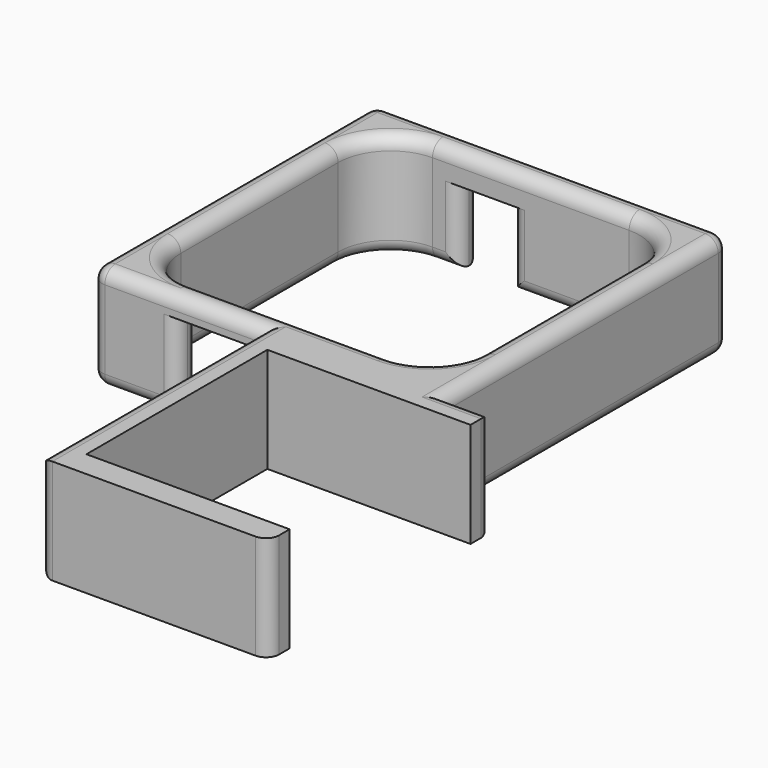
from build123d import *

# Parameters (mm, degrees)
F1_DEPTH      = 8
F2_W          = 13
F2_H          = 4
F2_W_2        = 8
F3_DEPTH      = 8
F4_DEPTH      = 5
F5_DEPTH      = 25
F6_DEPTH      = 3.5
F7_DEPTH      = 25
F8_R          = 8
F9_T1_DEPTH   = 52
F9_T3_DEPTH   = 12
F9_T5_DEPTH   = 12
F9_T7_DEPTH   = 33
F9_T9_DEPTH   = 50
F9_T11_DEPTH  = 8
F9_T13_DEPTH  = 16.5
F9_T15_DEPTH  = 19
F9_T17_DEPTH  = 30
F9_T19_DEPTH  = 50
F9_T21_DEPTH  = 16
F9_T23_DEPTH  = 24
F9_T25_DEPTH  = 17.8746859277
F9_T27_DEPTH  = 18
F9_T29_DEPTH  = 11
F9_T31_DEPTH  = 49.5
F9_T33_DEPTH  = 47.5
F9_T35_DEPTH  = 26
F9_T37_DEPTH  = 9
F9_T39_DEPTH  = 30
F9_T41_DEPTH  = 23
F9_T43_DEPTH  = 14
F9_S47_W      = 2.04
F9_S47_H      = 2.04
F9_T48_DEPTH  = 2.04
F9_S53_W      = 2.04
F9_S53_H      = 2.04
F9_T54_DEPTH  = 2.04
F9_S59_W      = 2.04
F9_S59_H      = 2.04
F9_T60_DEPTH  = 2.04
F9_S65_W      = 2.04
F9_S65_H      = 2.04
F9_T66_DEPTH  = 2.04
F9_S71_W      = 2.04
F9_S71_H      = 2.04
F9_T72_DEPTH  = 2.04
F9_S77_W      = 2.04
F9_S77_H      = 2.04
F9_T78_DEPTH  = 2.04
F9_S83_W      = 2.04
F9_S83_H      = 2.04
F9_T84_DEPTH  = 2.04
F9_T88_ANGLE  = 90
F9_T90_ANGLE  = 150.9012204259
F9_T92_ANGLE  = 90
F9_T94_ANGLE  = 90
F9_T96_ANGLE  = 90
F9_T98_ANGLE  = 90
F9_T100_ANGLE = 90
F9_T102_ANGLE = 90
F9_T107_DEPTH = 12
F9_T111_DEPTH = 57
F9_T119_DEPTH = 57
F9_T124_DEPTH = 12
F9_T131_DEPTH = 16.5
F9_T136_DEPTH = 13
F9_T143_DEPTH = 16.5
F9_T148_DEPTH = 13
F9_T155_DEPTH = 29
F9_T159_DEPTH = 47.5


# Not quite as in the source:
# - a fillet or chamfer that OpenCascade refuses, or shapes differently, is made with other operations: its cross-section is extruded or revolved along the edge and cut away or added


with BuildPart() as f1:
    # F0 (on Top) → F1 (new body, symmetric)
    with BuildSketch(Plane.XY):
        Polygon((29.4704200836, 10.5355388032), (29.4704200836, 14.5355388032), (-5.5295799164, 14.5355388032), (-5.5295799164, -27.9644611968), (29.4704200836, -27.9644611968), (29.4704200836, -23.9644611968), (27.4704200836, -23.9644611968), (-1.5295799164, -23.9644611968), (-1.5295799164, 10.5355388032), (27.4704200836, 10.5355388032), align=None)
    extrude(amount=F1_DEPTH, both=True)

    # F2 (on Top) → F3 (join, symmetric)
    with BuildSketch(Plane.XY):
        Polygon((-27.5295799164, 18.5355388032), (-27.5295799164, 64.5355388032), (-15.5295799164, 64.5355388032), (-15.5295799164, 68.5355388032), (-31.5295799164, 68.5355388032), (-31.5295799164, 14.5355388032), (-18.5295799164, 14.5355388032), (-18.5295799164, 18.5355388032), align=None)
        Polygon((-7.5295799164, 68.5355388032), (-7.5295799164, 64.5355388032), (18.4704200836, 64.5355388032), (18.4704200836, 18.5355388032), (-5.5295799164, 18.5355388032), (-5.5295799164, 14.5355388032), (22.4704200836, 14.5355388032), (22.4704200836, 68.5355388032), align=None)
        with Locations((-12.0295799164, 16.5355388032)):
            Rectangle(F2_W, F2_H)
        with Locations((-11.5295799164, 66.5355388032)):
            Rectangle(F2_W_2, F2_H)
    extrude(amount=F3_DEPTH, both=True)

    # F2 (on Top) → F4 (cut, symmetric)
    with BuildSketch(Plane.XY):
        with Locations((-12.0295799164, 16.5355388032)):
            Rectangle(F2_W, F2_H)
    extrude(amount=F4_DEPTH, both=True, mode=Mode.SUBTRACT)

    # F2 (on Top) → F5 (cut)
    with BuildSketch(Plane.XY):
        with Locations((-12.0295799164, 16.5355388032)):
            Rectangle(F2_W, F2_H)
    extrude(amount=-F5_DEPTH, mode=Mode.SUBTRACT)

    # F2 (on Top) → F6 (cut, symmetric)
    with BuildSketch(Plane.XY):
        with Locations((-11.5295799164, 66.5355388032)):
            Rectangle(F2_W_2, F2_H)
    extrude(amount=F6_DEPTH, both=True, mode=Mode.SUBTRACT)

    # F2 (on Top) → F7 (cut)
    with BuildSketch(Plane.XY):
        with Locations((-11.5295799164, 66.5355388032)):
            Rectangle(F2_W_2, F2_H)
    extrude(amount=-F7_DEPTH, mode=Mode.SUBTRACT)

    # F8
    f8_edges = [f1.edges().sort_by_distance(p)[0] for p in [
        (-27.52958, 64.535539, 0),
        (18.47042, 64.535539, 0),
        (-27.52958, 18.535539, 0),
        (18.47042, 18.535539, 0),
    ]]
    fillet(f8_edges, radius=F8_R)

    # F9: fillet of radius 2 on 44 edges, made by hand

    # F9_s2 → F9_t1 (cut)
    with BuildSketch(Plane.XZ.offset(-66.5355388032)):
        with BuildLine():
            ThreePointArc((20.4704200836, 8), (21.884633646, 7.4142135624), (22.4704200836, 6))
            Line((22.4704200836, 6), (22.4704200836, 8))
            Line((22.4704200836, 8), (20.4704200836, 8))
        make_face()
        with BuildLine():
            ThreePointArc((20.4704200836, -8), (21.884633646, -7.4142135624), (22.4704200836, -6))
            Line((22.4704200836, -6), (22.4704200836, -8))
            Line((22.4704200836, -8), (20.4704200836, -8))
        make_face()
    extrude(amount=F9_T1_DEPTH, mode=Mode.SUBTRACT)

    # F9_s4 → F9_t3 (cut)
    with BuildSketch(Plane.YZ.offset(22.4704200836)):
        with BuildLine():
            ThreePointArc((12.5355388032, 8), (13.9497523656, 7.4142135624), (14.5355388032, 6))
            Line((14.5355388032, 6), (14.5355388032, 8))
            Line((14.5355388032, 8), (12.5355388032, 8))
        make_face()
        with BuildLine():
            ThreePointArc((12.5355388032, -8), (13.9497523656, -7.4142135624), (14.5355388032, -6))
            Line((14.5355388032, -6), (14.5355388032, -8))
            Line((14.5355388032, -8), (12.5355388032, -8))
        make_face()
    extrude(amount=F9_T3_DEPTH, mode=Mode.SUBTRACT)

    # F9_s6 → F9_t5 (cut)
    with BuildSketch(Plane.XY.offset(-6)):
        with BuildLine():
            ThreePointArc((20.4704200836, 68.5355388032), (21.884633646, 67.9497523656), (22.4704200836, 66.5355388032))
            Line((22.4704200836, 66.5355388032), (22.4704200836, 68.5355388032))
            Line((22.4704200836, 68.5355388032), (20.4704200836, 68.5355388032))
        make_face()
        with BuildLine():
            ThreePointArc((-29.5295799164, 68.5355388032), (-30.9437934788, 67.9497523656), (-31.5295799164, 66.5355388032))
            Line((-31.5295799164, 66.5355388032), (-31.5295799164, 68.5355388032))
            Line((-31.5295799164, 68.5355388032), (-29.5295799164, 68.5355388032))
        make_face()
        with BuildLine():
            ThreePointArc((-31.5295799164, 16.5355388032), (-30.9437934788, 15.1213252408), (-29.5295799164, 14.5355388032))
            Line((-29.5295799164, 14.5355388032), (-31.5295799164, 14.5355388032))
            Line((-31.5295799164, 14.5355388032), (-31.5295799164, 16.5355388032))
        make_face()
    extrude(amount=F9_T5_DEPTH, mode=Mode.SUBTRACT)

    # F9_s8 → F9_t7 (cut)
    with BuildSketch(Plane.YZ.offset(-12.5295799164)):
        with BuildLine():
            ThreePointArc((68.5355388032, -6), (67.9497523656, -7.4142135624), (66.5355388032, -8))
            Line((66.5355388032, -8), (68.5355388032, -8))
            Line((68.5355388032, -8), (68.5355388032, -6))
        make_face()
    extrude(amount=F9_T7_DEPTH, mode=Mode.SUBTRACT)

    # F9_s10 → F9_t9 (cut)
    with BuildSketch(Plane.YZ.offset(-29.5295799164)):
        with BuildLine():
            ThreePointArc((68.5355388032, 6), (67.9497523656, 7.4142135624), (66.5355388032, 8))
            Line((66.5355388032, 8), (68.5355388032, 8))
            Line((68.5355388032, 8), (68.5355388032, 6))
        make_face()
    extrude(amount=F9_T9_DEPTH, mode=Mode.SUBTRACT)

    # F9_s12 → F9_t11 (cut)
    with BuildSketch(Plane.YZ.offset(-15.5295799164)):
        with BuildLine():
            ThreePointArc((68.5355388032, 5.5), (67.9497523656, 4.0857864376), (66.5355388032, 3.5))
            Line((66.5355388032, 3.5), (68.5355388032, 3.5))
            Line((68.5355388032, 3.5), (68.5355388032, 5.5))
        make_face()
    extrude(amount=F9_T11_DEPTH, mode=Mode.SUBTRACT)

    # F9_s14 → F9_t13 (cut)
    with BuildSketch(Plane.XY.offset(-13)):
        with BuildLine():
            ThreePointArc((-15.5295799164, 66.5355388032), (-16.115366354, 67.9497523656), (-17.5295799164, 68.5355388032))
            Line((-17.5295799164, 68.5355388032), (-15.5295799164, 68.5355388032))
            Line((-15.5295799164, 68.5355388032), (-15.5295799164, 66.5355388032))
        make_face()
        with BuildLine():
            ThreePointArc((-5.5295799164, 68.5355388032), (-6.9437934788, 67.9497523656), (-7.5295799164, 66.5355388032))
            Line((-7.5295799164, 66.5355388032), (-7.5295799164, 68.5355388032))
            Line((-7.5295799164, 68.5355388032), (-5.5295799164, 68.5355388032))
        make_face()
        with BuildLine():
            ThreePointArc((-5.5295799164, 64.5355388032), (-6.9437934788, 65.1213252408), (-7.5295799164, 66.5355388032))
            Line((-7.5295799164, 66.5355388032), (-7.5295799164, 64.5355388032))
            Line((-7.5295799164, 64.5355388032), (-5.5295799164, 64.5355388032))
        make_face()
        with BuildLine():
            ThreePointArc((-17.5295799164, 64.5355388032), (-16.115366354, 65.1213252408), (-15.5295799164, 66.5355388032))
            Line((-15.5295799164, 66.5355388032), (-15.5295799164, 64.5355388032))
            Line((-15.5295799164, 64.5355388032), (-17.5295799164, 64.5355388032))
        make_face()
    extrude(amount=F9_T13_DEPTH, mode=Mode.SUBTRACT)

    # F9_s16 → F9_t15 (cut)
    with BuildSketch(Plane.YZ.offset(-29.5295799164)):
        with BuildLine():
            ThreePointArc((66.5355388032, -8), (67.9497523656, -7.4142135624), (68.5355388032, -6))
            Line((68.5355388032, -6), (68.5355388032, -8))
            Line((68.5355388032, -8), (66.5355388032, -8))
        make_face()
    extrude(amount=F9_T15_DEPTH, mode=Mode.SUBTRACT)

    # F9_s18 → F9_t17 (cut)
    with BuildSketch(Plane.XZ.offset(-56.5355388032)):
        with BuildLine():
            ThreePointArc((-29.5295799164, -8), (-28.115366354, -7.4142135624), (-27.5295799164, -6))
            Line((-27.5295799164, -6), (-27.5295799164, -8))
            Line((-27.5295799164, -8), (-29.5295799164, -8))
        make_face()
        with BuildLine():
            ThreePointArc((20.4704200836, -8), (19.0562065212, -7.4142135624), (18.4704200836, -6))
            Line((18.4704200836, -6), (18.4704200836, -8))
            Line((18.4704200836, -8), (20.4704200836, -8))
        make_face()
        with BuildLine():
            ThreePointArc((-27.5295799164, 6), (-28.115366354, 7.4142135624), (-29.5295799164, 8))
            Line((-29.5295799164, 8), (-27.5295799164, 8))
            Line((-27.5295799164, 8), (-27.5295799164, 6))
        make_face()
        with BuildLine():
            ThreePointArc((20.4704200836, 8), (19.0562065212, 7.4142135624), (18.4704200836, 6))
            Line((18.4704200836, 6), (18.4704200836, 8))
            Line((18.4704200836, 8), (20.4704200836, 8))
        make_face()
    extrude(amount=F9_T17_DEPTH, mode=Mode.SUBTRACT)

    # F9_s20 → F9_t19 (cut)
    with BuildSketch(Plane.XZ.offset(-66.5355388032)):
        with BuildLine():
            ThreePointArc((-29.5295799164, -8), (-30.9437934788, -7.4142135624), (-31.5295799164, -6))
            Line((-31.5295799164, -6), (-31.5295799164, -8))
            Line((-31.5295799164, -8), (-29.5295799164, -8))
        make_face()
        with BuildLine():
            ThreePointArc((-31.5295799164, 6), (-30.9437934788, 7.4142135624), (-29.5295799164, 8))
            Line((-29.5295799164, 8), (-31.5295799164, 8))
            Line((-31.5295799164, 8), (-31.5295799164, 6))
        make_face()
    extrude(amount=F9_T19_DEPTH, mode=Mode.SUBTRACT)

    # F9_s22 → F9_t21 (cut)
    with BuildSketch(Plane.YZ.offset(-29.5295799164)):
        with BuildLine():
            ThreePointArc((16.5355388032, -8), (15.1213252408, -7.4142135624), (14.5355388032, -6))
            Line((14.5355388032, -6), (14.5355388032, -8))
            Line((14.5355388032, -8), (16.5355388032, -8))
        make_face()
    extrude(amount=F9_T21_DEPTH, mode=Mode.SUBTRACT)

    # F9_s24 → F9_t23 (cut)
    with BuildSketch(Plane.YZ.offset(-29.5295799164)):
        with BuildLine():
            ThreePointArc((14.5355388032, 6), (15.1213252408, 7.4142135624), (16.5355388032, 8))
            Line((16.5355388032, 8), (14.5355388032, 8))
            Line((14.5355388032, 8), (14.5355388032, 6))
        make_face()
    extrude(amount=F9_T23_DEPTH, mode=Mode.SUBTRACT)

    # F9_s26 → F9_t25 (cut)
    with BuildSketch(Plane.XY.offset(-12.8746859277)):
        with BuildLine():
            ThreePointArc((-20.3295799164, 18.5756393063), (-19.046340219, 17.9273052186), (-18.5295799164, 16.5856644321))
            Line((-18.5295799164, 16.5856644321), (-18.3295799164, 16.5856644321))
            Line((-18.3295799164, 16.5856644321), (-18.3295799164, 18.5355388032))
            Line((-18.3295799164, 18.5355388032), (-18.5295799164, 18.7355388032))
            ThreePointArc((-18.5295799164, 18.7355388032), (-19.5295799164, 18.7355388032), (-20.3095799164, 18.7746367938))
            Line((-20.3095799164, 18.7746367938), (-20.3295799164, 18.5756393063))
        make_face()
    extrude(amount=F9_T25_DEPTH, mode=Mode.SUBTRACT)

    # F9_s28 → F9_t27 (cut)
    with BuildSketch(Plane.XY.offset(-13)):
        with BuildLine():
            ThreePointArc((-20.5295799164, 14.5355388032), (-19.115366354, 15.1213252408), (-18.5295799164, 16.5355388032))
            Line((-18.5295799164, 16.5355388032), (-18.5295799164, 14.5355388032))
            Line((-18.5295799164, 14.5355388032), (-20.5295799164, 14.5355388032))
        make_face()
    extrude(amount=F9_T27_DEPTH, mode=Mode.SUBTRACT)

    # F9_s30 → F9_t29 (cut)
    with BuildSketch(Plane.XY.offset(-6)):
        with BuildLine():
            ThreePointArc((-3.5295799164, 18.5355388032), (-4.9437934788, 17.9497523656), (-5.5295799164, 16.5355388032))
            Line((-5.5295799164, 16.5355388032), (-5.5295799164, 18.5355388032))
            Line((-5.5295799164, 18.5355388032), (-3.5295799164, 18.5355388032))
        make_face()
    extrude(amount=F9_T29_DEPTH, mode=Mode.SUBTRACT)

    # F9_s32 → F9_t31 (cut)
    with BuildSketch(Plane.XZ.offset(-16.5355388032)):
        with BuildLine():
            ThreePointArc((-3.5295799164, -8), (-4.9437934788, -7.4142135624), (-5.5295799164, -6))
            Line((-5.5295799164, -6), (-5.5295799164, -8))
            Line((-5.5295799164, -8), (-3.5295799164, -8))
        make_face()
    extrude(amount=F9_T31_DEPTH, mode=Mode.SUBTRACT)

    # F9_s34 → F9_t33 (cut)
    with BuildSketch(Plane.XZ.offset(-14.5355388032)):
        with BuildLine():
            ThreePointArc((-3.5295799164, 8), (-4.9437934788, 7.4142135624), (-5.5295799164, 6))
            Line((-5.5295799164, 6), (-5.5295799164, 8))
            Line((-5.5295799164, 8), (-3.5295799164, 8))
        make_face()
    extrude(amount=F9_T33_DEPTH, mode=Mode.SUBTRACT)

    # F9_s36 → F9_t35 (cut)
    with BuildSketch(Plane.XY.offset(-13)):
        with BuildLine():
            ThreePointArc((27.4704200836, -27.9644611968), (28.884633646, -27.3786747592), (29.4704200836, -25.9644611968))
            Line((29.4704200836, -25.9644611968), (29.4704200836, -27.9644611968))
            Line((29.4704200836, -27.9644611968), (27.4704200836, -27.9644611968))
        make_face()
        with BuildLine():
            ThreePointArc((-5.5295799164, -25.9644611968), (-4.9437934788, -27.3786747592), (-3.5295799164, -27.9644611968))
            Line((-3.5295799164, -27.9644611968), (-5.5295799164, -27.9644611968))
            Line((-5.5295799164, -27.9644611968), (-5.5295799164, -25.9644611968))
        make_face()
        with BuildLine():
            ThreePointArc((29.4704200836, 12.5355388032), (28.884633646, 13.9497523656), (27.4704200836, 14.5355388032))
            Line((27.4704200836, 14.5355388032), (29.4704200836, 14.5355388032))
            Line((29.4704200836, 14.5355388032), (29.4704200836, 12.5355388032))
        make_face()
    extrude(amount=F9_T35_DEPTH, mode=Mode.SUBTRACT)

    # F9_s38 → F9_t37 (cut)
    with BuildSketch(Plane.YZ.offset(-19.5295799164)):
        with BuildLine():
            ThreePointArc((66.5355388032, -8), (65.1213252408, -7.4142135624), (64.5355388032, -6))
            Line((64.5355388032, -6), (64.5355388032, -8))
            Line((64.5355388032, -8), (66.5355388032, -8))
        make_face()
    extrude(amount=F9_T37_DEPTH, mode=Mode.SUBTRACT)

    # F9_s40 → F9_t39 (cut)
    with BuildSketch(Plane.YZ.offset(-19.5295799164)):
        with BuildLine():
            ThreePointArc((64.5355388032, 6), (65.1213252408, 7.4142135624), (66.5355388032, 8))
            Line((66.5355388032, 8), (64.5355388032, 8))
            Line((64.5355388032, 8), (64.5355388032, 6))
        make_face()
        with BuildLine():
            ThreePointArc((18.5355388032, 6), (17.9497523656, 7.4142135624), (16.5355388032, 8))
            Line((16.5355388032, 8), (18.5355388032, 8))
            Line((18.5355388032, 8), (18.5355388032, 6))
        make_face()
    extrude(amount=F9_T39_DEPTH, mode=Mode.SUBTRACT)

    # F9_s42 → F9_t41 (cut)
    with BuildSketch(Plane.YZ.offset(-12.5295799164)):
        with BuildLine():
            ThreePointArc((64.5355388032, -6), (65.1213252408, -7.4142135624), (66.5355388032, -8))
            Line((66.5355388032, -8), (64.5355388032, -8))
            Line((64.5355388032, -8), (64.5355388032, -6))
        make_face()
    extrude(amount=F9_T41_DEPTH, mode=Mode.SUBTRACT)

    # F9_s44 → F9_t43 (cut)
    with BuildSketch(Plane.YZ.offset(-3.5295799164)):
        with BuildLine():
            ThreePointArc((18.5355388032, -6), (17.9497523656, -7.4142135624), (16.5355388032, -8))
            Line((16.5355388032, -8), (18.5355388032, -8))
            Line((18.5355388032, -8), (18.5355388032, -6))
        make_face()
    extrude(amount=F9_T43_DEPTH, mode=Mode.SUBTRACT)


with BuildPart() as f9_tool46:
    # F9_s47 → F9_t48 (new body)
    with BuildSketch(Plane.YZ.offset(20.4704200836)):
        with Locations((67.5555388032, 7.02)):
            Rectangle(F9_S47_W, F9_S47_H)
    extrude(amount=F9_T48_DEPTH)

    # F9_s49 → F9_t50 (revolve, cut)
    with BuildSketch(Plane(origin=(20.4704200836, 66.5355388032, 6), x_dir=(0, -0.7071067812, -0.7071067812), z_dir=(0, -0.7071067812, 0.7071067812))):
        with BuildLine():
            ThreePointArc((0, -2), (2, 0), (0, 2))
            Line((0, 2), (0, -2))
        make_face()
    revolve(axis=Axis((20.4704200836, 66.5355388032, 6), (1, 0, 0)), mode=Mode.SUBTRACT)


with BuildPart() as f1_1:
    add(f1.part)

    # F9_t45: cut F9_tool46
    add(f9_tool46.part, mode=Mode.SUBTRACT)


with BuildPart() as f9_tool52:
    # F9_s53 → F9_t54 (new body)
    with BuildSketch(Plane.YZ.offset(20.4704200836)):
        with Locations((67.5555388032, -7.02)):
            Rectangle(F9_S53_W, F9_S53_H)
    extrude(amount=F9_T54_DEPTH)

    # F9_s55 → F9_t56 (revolve, cut)
    with BuildSketch(Plane(origin=(20.4704200836, 66.5355388032, -6), x_dir=(0, -0.7071067812, 0.7071067812), z_dir=(0, 0.7071067812, 0.7071067812))):
        with BuildLine():
            ThreePointArc((0, -2), (2, 0), (0, 2))
            Line((0, 2), (0, -2))
        make_face()
    revolve(axis=Axis((20.4704200836, 66.5355388032, -6), (1, 0, 0)), mode=Mode.SUBTRACT)


with BuildPart() as f1_2:
    add(f1_1.part)

    # F9_t51: cut F9_tool52
    add(f9_tool52.part, mode=Mode.SUBTRACT)


with BuildPart() as f9_tool58:
    # F9_s59 → F9_t60 (new body)
    with BuildSketch(Plane.XY.offset(6)):
        with Locations((-30.5495799164, 67.5555388032)):
            Rectangle(F9_S59_W, F9_S59_H)
    extrude(amount=F9_T60_DEPTH)

    # F9_s61 → F9_t62 (revolve, cut)
    with BuildSketch(Plane(origin=(-29.5295799164, 66.5355388032, 6), x_dir=(0.7071067812, -0.7071067812, 0), z_dir=(-0.7071067812, -0.7071067812, 0))):
        with BuildLine():
            ThreePointArc((0, -2), (2, 0), (0, 2))
            Line((0, 2), (0, -2))
        make_face()
    revolve(axis=Axis((-29.5295799164, 66.5355388032, 6), (0, 0, 1)), mode=Mode.SUBTRACT)


with BuildPart() as f1_3:
    add(f1_2.part)

    # F9_t57: cut F9_tool58
    add(f9_tool58.part, mode=Mode.SUBTRACT)


with BuildPart() as f9_tool64:
    # F9_s65 → F9_t66 (new body)
    with BuildSketch(Plane.XY.offset(-6)):
        with Locations((-30.5495799164, 67.5555388032)):
            Rectangle(F9_S65_W, F9_S65_H)
    extrude(amount=-F9_T66_DEPTH)

    # F9_s67 → F9_t68 (revolve, cut)
    with BuildSketch(Plane(origin=(-29.5295799164, 66.5355388032, -6), x_dir=(0.7071067812, -0.7071067812, 0), z_dir=(0.7071067812, 0.7071067812, 0))):
        with BuildLine():
            ThreePointArc((0, -2), (2, 0), (0, 2))
            Line((0, 2), (0, -2))
        make_face()
    revolve(axis=Axis((-29.5295799164, 66.5355388032, -6), (0, 0, -1)), mode=Mode.SUBTRACT)


with BuildPart() as f1_4:
    add(f1_3.part)

    # F9_t63: cut F9_tool64
    add(f9_tool64.part, mode=Mode.SUBTRACT)


with BuildPart() as f9_tool70:
    # F9_s71 → F9_t72 (new body)
    with BuildSketch(Plane.XY.offset(-6)):
        with Locations((-30.5495799164, 15.5155388032)):
            Rectangle(F9_S71_W, F9_S71_H)
    extrude(amount=-F9_T72_DEPTH)

    # F9_s73 → F9_t74 (revolve, cut)
    with BuildSketch(Plane(origin=(-29.5295799164, 16.5355388032, -6), x_dir=(0.7071067812, 0.7071067812, 0), z_dir=(-0.7071067812, 0.7071067812, 0))):
        with BuildLine():
            ThreePointArc((0, -2), (2, 0), (0, 2))
            Line((0, 2), (0, -2))
        make_face()
    revolve(axis=Axis((-29.5295799164, 16.5355388032, -6), (0, 0, -1)), mode=Mode.SUBTRACT)


with BuildPart() as f1_5:
    add(f1_4.part)

    # F9_t69: cut F9_tool70
    add(f9_tool70.part, mode=Mode.SUBTRACT)


with BuildPart() as f9_tool76:
    # F9_s77 → F9_t78 (new body)
    with BuildSketch(Plane.XZ.offset(-16.5355388032)):
        with Locations((-30.5495799164, 7.02)):
            Rectangle(F9_S77_W, F9_S77_H)
    extrude(amount=F9_T78_DEPTH)

    # F9_s79 → F9_t80 (revolve, cut)
    with BuildSketch(Plane(origin=(-29.5295799164, 16.5355388032, 6), x_dir=(0.7071067812, 0, -0.7071067812), z_dir=(-0.7071067812, 0, -0.7071067812))):
        with BuildLine():
            ThreePointArc((0, -2), (2, 0), (0, 2))
            Line((0, 2), (0, -2))
        make_face()
    revolve(axis=Axis((-29.5295799164, 16.5355388032, 6), (0, -1, 0)), mode=Mode.SUBTRACT)


with BuildPart() as f1_6:
    add(f1_5.part)

    # F9_t75: cut F9_tool76
    add(f9_tool76.part, mode=Mode.SUBTRACT)


with BuildPart() as f9_tool82:
    # F9_s83 → F9_t84 (new body)
    with BuildSketch(Plane.XZ.offset(-16.5355388032)):
        with Locations((-4.5495799164, -7.02)):
            Rectangle(F9_S83_W, F9_S83_H)
    extrude(amount=-F9_T84_DEPTH)

    # F9_s85 → F9_t86 (revolve, cut)
    with BuildSketch(Plane(origin=(-3.5295799164, 16.5355388032, -6), x_dir=(0.7071067812, 0, 0.7071067812), z_dir=(-0.7071067812, 0, 0.7071067812))):
        with BuildLine():
            ThreePointArc((0, -2), (2, 0), (0, 2))
            Line((0, 2), (0, -2))
        make_face()
    revolve(axis=Axis((-3.5295799164, 16.5355388032, -6), (0, 1, 0)), mode=Mode.SUBTRACT)


with BuildPart() as f1_7:
    add(f1_6.part)

    # F9_t81: cut F9_tool82
    add(f9_tool82.part, mode=Mode.SUBTRACT)

    # F9_s87 → F9_t88 (revolve, cut)
    with BuildSketch(Plane.XZ.offset(-56.5355388032)):
        with BuildLine():
            ThreePointArc((-29.5295799164, -8), (-28.115366354, -7.4142135624), (-27.5295799164, -6))
            Line((-27.5295799164, -6), (-27.5295799164, -8))
            Line((-27.5295799164, -8), (-29.5295799164, -8))
        make_face()
    revolve(axis=Axis((-19.5295799164, 56.5355388032, -8), (0, 0, -1)), revolution_arc=F9_T88_ANGLE, mode=Mode.SUBTRACT)

    # F9_s89 → F9_t90 (revolve, cut)
    with BuildSketch(Plane.XZ.offset(-26.5355388032)):
        with BuildLine():
            ThreePointArc((-29.5295799164, -8), (-28.115366354, -7.4142135624), (-27.5295799164, -6))
            Line((-27.5295799164, -6), (-27.5295799164, -8))
            Line((-27.5295799164, -8), (-29.5295799164, -8))
        make_face()
    revolve(axis=Axis((-19.5295799164, 26.5355388032, -8), (0, 0, 1)), revolution_arc=F9_T90_ANGLE, mode=Mode.SUBTRACT)

    # F9_s91 → F9_t92 (revolve, cut)
    with BuildSketch(Plane.XZ.offset(-56.5355388032)):
        with BuildLine():
            ThreePointArc((-27.5295799164, 6), (-28.115366354, 7.4142135624), (-29.5295799164, 8))
            Line((-29.5295799164, 8), (-27.5295799164, 8))
            Line((-27.5295799164, 8), (-27.5295799164, 6))
        make_face()
    revolve(axis=Axis((-19.5295799164, 56.5355388032, 8), (0, 0, -1)), revolution_arc=F9_T92_ANGLE, mode=Mode.SUBTRACT)

    # F9_s93 → F9_t94 (revolve, cut)
    with BuildSketch(Plane.XZ.offset(-26.5355388032)):
        with BuildLine():
            ThreePointArc((-27.5295799164, 6), (-28.115366354, 7.4142135624), (-29.5295799164, 8))
            Line((-29.5295799164, 8), (-27.5295799164, 8))
            Line((-27.5295799164, 8), (-27.5295799164, 6))
        make_face()
    revolve(axis=Axis((-19.5295799164, 26.5355388032, 8), (0, 0, 1)), revolution_arc=F9_T94_ANGLE, mode=Mode.SUBTRACT)

    # F9_s95 → F9_t96 (revolve, cut)
    with BuildSketch(Plane.XZ.offset(-26.5355388032)):
        with BuildLine():
            ThreePointArc((20.4704200836, 8), (19.0562065212, 7.4142135624), (18.4704200836, 6))
            Line((18.4704200836, 6), (18.4704200836, 8))
            Line((18.4704200836, 8), (20.4704200836, 8))
        make_face()
    revolve(axis=Axis((10.4704200836, 26.5355388032, 8), (0, 0, -1)), revolution_arc=F9_T96_ANGLE, mode=Mode.SUBTRACT)

    # F9_s97 → F9_t98 (revolve, cut)
    with BuildSketch(Plane.YZ.offset(10.4704200836)):
        with BuildLine():
            ThreePointArc((66.5355388032, 8), (65.1213252408, 7.4142135624), (64.5355388032, 6))
            Line((64.5355388032, 6), (64.5355388032, 8))
            Line((64.5355388032, 8), (66.5355388032, 8))
        make_face()
    revolve(axis=Axis((10.4704200836, 56.5355388032, 8), (0, 0, -1)), revolution_arc=F9_T98_ANGLE, mode=Mode.SUBTRACT)

    # F9_s99 → F9_t100 (revolve, cut)
    with BuildSketch(Plane.YZ.offset(10.4704200836)):
        with BuildLine():
            ThreePointArc((64.5355388032, -6), (65.1213252408, -7.4142135624), (66.5355388032, -8))
            Line((66.5355388032, -8), (64.5355388032, -8))
            Line((64.5355388032, -8), (64.5355388032, -6))
        make_face()
    revolve(axis=Axis((10.4704200836, 56.5355388032, -8), (0, 0, -1)), revolution_arc=F9_T100_ANGLE, mode=Mode.SUBTRACT)

    # F9_s101 → F9_t102 (revolve, cut)
    with BuildSketch(Plane.XZ.offset(-26.5355388032)):
        with BuildLine():
            ThreePointArc((20.4704200836, -8), (19.0562065212, -7.4142135624), (18.4704200836, -6))
            Line((18.4704200836, -6), (18.4704200836, -8))
            Line((18.4704200836, -8), (20.4704200836, -8))
        make_face()
    revolve(axis=Axis((10.4704200836, 26.5355388032, -8), (0, 0, -1)), revolution_arc=F9_T102_ANGLE, mode=Mode.SUBTRACT)


with BuildPart() as f9_tool105:
    # F9_s106 → F9_t107 (new body)
    with BuildSketch(Plane.YZ.offset(29.4704200836)):
        with BuildLine():
            ThreePointArc((12.5355388032, 8), (13.9497523656, 7.4142135624), (14.5355388032, 6))
            Line((14.5355388032, 6), (14.5355388032, 8))
            Line((14.5355388032, 8), (12.5355388032, 8))
        make_face()
    extrude(amount=-F9_T107_DEPTH)

    split(bisect_by=Plane.YZ.offset(22.4704200836), keep=Keep.BOTTOM)


with BuildPart() as f9_tool109:
    # F9_s110 → F9_t111 (new body)
    with BuildSketch(Plane.XZ.offset(-9.5355388032)):
        with BuildLine():
            ThreePointArc((20.4704200836, 8), (21.884633646, 7.4142135624), (22.4704200836, 6))
            Line((22.4704200836, 6), (22.4704200836, 8))
            Line((22.4704200836, 8), (20.4704200836, 8))
        make_face()
    extrude(amount=-F9_T111_DEPTH)

    split(bisect_by=Plane.XZ.offset(-14.5355388032), keep=Keep.TOP)

    split(bisect_by=Plane.XZ.offset(-10.5355388032), keep=Keep.BOTTOM)


with BuildPart() as f9_tool105_1:
    add(f9_tool105.part)

    # F9_t114: intersect F9_tool109
    add(f9_tool109.part, mode=Mode.INTERSECT)


with BuildPart() as f1_8:
    add(f1_7.part)

    # F9_t103: cut F9_tool105
    add(f9_tool105_1.part, mode=Mode.SUBTRACT)


with BuildPart() as f9_tool117:
    # F9_s118 → F9_t119 (new body)
    with BuildSketch(Plane.XZ.offset(-9.5355388032)):
        with BuildLine():
            ThreePointArc((20.4704200836, -8), (21.884633646, -7.4142135624), (22.4704200836, -6))
            Line((22.4704200836, -6), (22.4704200836, -8))
            Line((22.4704200836, -8), (20.4704200836, -8))
        make_face()
    extrude(amount=-F9_T119_DEPTH)

    split(bisect_by=Plane.XZ.offset(-14.5355388032), keep=Keep.TOP)

    split(bisect_by=Plane.XZ.offset(-10.5355388032), keep=Keep.BOTTOM)


with BuildPart() as f9_tool122:
    # F9_s123 → F9_t124 (new body)
    with BuildSketch(Plane.YZ.offset(29.4704200836)):
        with BuildLine():
            ThreePointArc((12.5355388032, -8), (13.9497523656, -7.4142135624), (14.5355388032, -6))
            Line((14.5355388032, -6), (14.5355388032, -8))
            Line((14.5355388032, -8), (12.5355388032, -8))
        make_face()
    extrude(amount=-F9_T124_DEPTH)

    split(bisect_by=Plane.YZ.offset(22.4704200836), keep=Keep.BOTTOM)


with BuildPart() as f9_tool117_1:
    add(f9_tool117.part)

    # F9_t126: intersect F9_tool122
    add(f9_tool122.part, mode=Mode.INTERSECT)


with BuildPart() as f1_9:
    add(f1_8.part)

    # F9_t115: cut F9_tool117
    add(f9_tool117_1.part, mode=Mode.SUBTRACT)


with BuildPart() as f9_tool129:
    # F9_s130 → F9_t131 (new body)
    with BuildSketch(Plane.XY.offset(8.5)):
        with BuildLine():
            ThreePointArc((-5.5295799164, 68.5355388032), (-6.9437934788, 67.9497523656), (-7.5295799164, 66.5355388032))
            Line((-7.5295799164, 66.5355388032), (-7.5295799164, 68.5355388032))
            Line((-7.5295799164, 68.5355388032), (-5.5295799164, 68.5355388032))
        make_face()
    extrude(amount=-F9_T131_DEPTH)

    split(bisect_by=Plane.XY.offset(8), keep=Keep.BOTTOM)

    split(bisect_by=Plane.XY.offset(3.5), keep=Keep.TOP)


with BuildPart() as f9_tool134:
    # F9_s135 → F9_t136 (new body)
    with BuildSketch(Plane.YZ.offset(-2.5295799164)):
        with BuildLine():
            ThreePointArc((68.5355388032, 5.5), (67.9497523656, 4.0857864376), (66.5355388032, 3.5))
            Line((66.5355388032, 3.5), (68.5355388032, 3.5))
            Line((68.5355388032, 3.5), (68.5355388032, 5.5))
        make_face()
    extrude(amount=-F9_T136_DEPTH)

    split(bisect_by=Plane.YZ.offset(-7.5295799164), keep=Keep.TOP)


with BuildPart() as f9_tool129_1:
    add(f9_tool129.part)

    # F9_t138: intersect F9_tool134
    add(f9_tool134.part, mode=Mode.INTERSECT)


with BuildPart() as f1_10:
    add(f1_9.part)

    # F9_t127: cut F9_tool129
    add(f9_tool129_1.part, mode=Mode.SUBTRACT)


with BuildPart() as f9_tool141:
    # F9_s142 → F9_t143 (new body)
    with BuildSketch(Plane.XY.offset(8.5)):
        with BuildLine():
            ThreePointArc((-15.5295799164, 66.5355388032), (-16.115366354, 67.9497523656), (-17.5295799164, 68.5355388032))
            Line((-17.5295799164, 68.5355388032), (-15.5295799164, 68.5355388032))
            Line((-15.5295799164, 68.5355388032), (-15.5295799164, 66.5355388032))
        make_face()
    extrude(amount=-F9_T143_DEPTH)

    split(bisect_by=Plane.XY.offset(8), keep=Keep.BOTTOM)

    split(bisect_by=Plane.XY.offset(3.5), keep=Keep.TOP)


with BuildPart() as f9_tool146:
    # F9_s147 → F9_t148 (new body)
    with BuildSketch(Plane.YZ.offset(-7.5295799164)):
        with BuildLine():
            ThreePointArc((68.5355388032, 5.5), (67.9497523656, 4.0857864376), (66.5355388032, 3.5))
            Line((66.5355388032, 3.5), (68.5355388032, 3.5))
            Line((68.5355388032, 3.5), (68.5355388032, 5.5))
        make_face()
    extrude(amount=-F9_T148_DEPTH)

    split(bisect_by=Plane.YZ.offset(-15.5295799164), keep=Keep.BOTTOM)


with BuildPart() as f9_tool141_1:
    add(f9_tool141.part)

    # F9_t150: intersect F9_tool146
    add(f9_tool146.part, mode=Mode.INTERSECT)


with BuildPart() as f1_11:
    add(f1_10.part)

    # F9_t139: cut F9_tool141
    add(f9_tool141_1.part, mode=Mode.SUBTRACT)


with BuildPart() as f9_tool153:
    # F9_s154 → F9_t155 (new body)
    with BuildSketch(Plane.YZ.offset(-29.5295799164)):
        with BuildLine():
            ThreePointArc((14.5355388032, 6), (15.1213252408, 7.4142135624), (16.5355388032, 8))
            Line((16.5355388032, 8), (14.5355388032, 8))
            Line((14.5355388032, 8), (14.5355388032, 6))
        make_face()
    extrude(amount=F9_T155_DEPTH)

    split(bisect_by=Plane.YZ.offset(-5.5295799164), keep=Keep.TOP)


with BuildPart() as f9_tool157:
    # F9_s158 → F9_t159 (new body)
    with BuildSketch(Plane.XZ.offset(-19.5355388032)):
        with BuildLine():
            ThreePointArc((-3.5295799164, 8), (-4.9437934788, 7.4142135624), (-5.5295799164, 6))
            Line((-5.5295799164, 6), (-5.5295799164, 8))
            Line((-5.5295799164, 8), (-3.5295799164, 8))
        make_face()
    extrude(amount=F9_T159_DEPTH)

    split(bisect_by=Plane.XZ.offset(-18.5355388032), keep=Keep.TOP)

    split(bisect_by=Plane.XZ.offset(-14.5355388032), keep=Keep.BOTTOM)


with BuildPart() as f9_tool153_1:
    add(f9_tool153.part)

    # F9_t162: intersect F9_tool157
    add(f9_tool157.part, mode=Mode.INTERSECT)


with BuildPart() as f1_12:
    add(f1_11.part)

    # F9_t151: cut F9_tool153
    add(f9_tool153_1.part, mode=Mode.SUBTRACT)


solid = f1_12.part
